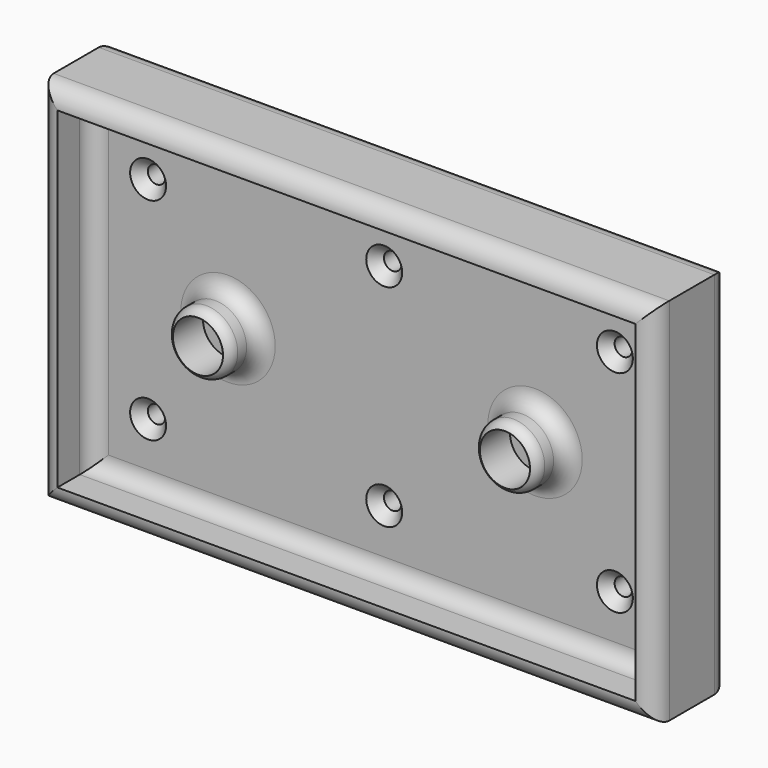
from build123d import *

# Parameters (mm, degrees)
F0_W            = 98.3085063696
F0_H            = 59.0165173113
F0_W_2          = 92.3085063696
F0_H_2          = 53.0165173113
F1_DEPTH        = 8
F2_DEPTH        = 15
F3_R            = 5
F3_R_2          = 4
F4_DEPTH        = 6
F5_R            = 2.54
F6_R            = 3
F7_R            = 2.99999
F10_D           = 2.794
F10_CSINK_D     = 5.7404
F10_CSINK_ANGLE = 82


# Not quite as in the source:
# - a fillet or chamfer that OpenCascade refuses, or shapes differently, is made with other operations: its cross-section is extruded or revolved along the edge and cut away or added
# - a fillet or chamfer is up to 0.001 mm smaller than in the source, because OpenCascade refuses the exact size


with BuildPart() as f1:
    # F0 (on Front) → F1 (new body)
    with BuildSketch(Plane.XZ):
        Rectangle(F0_W, F0_H)
        Rectangle(F0_W_2, F0_H_2, mode=Mode.SUBTRACT)
        Rectangle(F0_W_2, F0_H_2)
    extrude(amount=F1_DEPTH)

    # F0 (on Front) → F2 (join)
    with BuildSketch(Plane.XZ):
        Rectangle(F0_W, F0_H)
        Rectangle(F0_W_2, F0_H_2, mode=Mode.SUBTRACT)
    extrude(amount=F2_DEPTH)

    # F3 (on face) → F4 (join)
    with BuildSketch(Plane.XZ.offset(8)):
        with Locations((-24.5116613805, 0)):
            Circle(F3_R)
        with Locations((-24.5116613805, 0)):
            Circle(F3_R_2, mode=Mode.SUBTRACT)
        with Locations((24.5116613805, 0)):
            Circle(F3_R)
        with Locations((24.5116613805, 0)):
            Circle(F3_R_2, mode=Mode.SUBTRACT)
    extrude(amount=F4_DEPTH)

    # F5
    f5_edges = [f1.edges().sort_by_distance(p)[0] for p in [
        (-29.511661, -8, 0),
        (19.511661, -8, 0),
        (0, -8, -26.508259),
        (46.154253, -8, 0),
        (-46.154253, -8, 0),
        (0, -8, 26.508259),
    ]]
    fillet(f5_edges, radius=F5_R)

    # F6
    f6_edges = [f1.edges().sort_by_distance(p)[0] for p in [
        (0, 0, 29.508259),
        (49.154253, 0, 0),
        (0, 0, -29.508259),
        (-49.154253, 0, 0),
    ]]
    fillet(f6_edges, radius=F6_R)

    # F7 (radius 3 in the source; OpenCascade refuses exactly that, so slightly less here)
    f7_edges = [f1.edges().sort_by_distance(p)[0] for p in [
        (0, -15, -29.508259),
        (49.154253, -15, 0),
        (-49.154253, -15, 0),
        (0, -15, 29.508259),
    ]]
    fillet(f7_edges, radius=F7_R)

    # F8: fillet of radius 2 on 2 edges, made by hand

    # F8_s1 → F8_t2 (revolve, cut)
    with BuildSketch(Plane.XY):
        with BuildLine():
            ThreePointArc((29.5120613805, -12.2673917434), (29.2440686279, -13.2678330874), (28.5118614771, -14.0003463544))
            Line((28.5118614771, -14.0003463544), (28.6119780552, -14.1736418155))
            ThreePointArc((28.6119780552, -14.1736418155), (29.0117614288, -14.2001365685), (29.5116613805, -14.2001365685))
            Line((29.5116613805, -14.2001365685), (29.7117979491, -14))
            ThreePointArc((29.7117979491, -14), (29.7117979491, -13.1336958717), (29.7121979491, -12.2673917434))
            Line((29.7121979491, -12.2673917434), (29.5120613805, -12.2673917434))
        make_face()
    revolve(axis=Axis((24.5116613805, -14, 0), (0, -1, 0)), mode=Mode.SUBTRACT)

    # F8_s3 → F8_t4 (revolve, cut)
    with BuildSketch(Plane.XY):
        with BuildLine():
            ThreePointArc((-19.5112613805, -12.2673917434), (-19.7792541332, -13.2678330874), (-20.511461284, -14.0003463544))
            Line((-20.511461284, -14.0003463544), (-20.4113447058, -14.1736418155))
            ThreePointArc((-20.4113447058, -14.1736418155), (-20.0115613323, -14.2001365685), (-19.5116613805, -14.2001365685))
            Line((-19.5116613805, -14.2001365685), (-19.311524812, -14))
            ThreePointArc((-19.311524812, -14), (-19.311524812, -13.1336958717), (-19.311124812, -12.2673917434))
            Line((-19.311124812, -12.2673917434), (-19.5112613805, -12.2673917434))
        make_face()
    revolve(axis=Axis((-24.5116613805, -14, 0), (0, -1, 0)), mode=Mode.SUBTRACT)

    # F10 (through all)
    with Locations(Plane.XZ.offset(8)):
        with Locations((37.2699052095, 16.8491732329), (37.2699052095, -16.8491732329), (0.4332323442, -16.7640619911), (0.4332323442, 16.9342844747), (-37.2699052095, 16.8491732329), (-37.2699052095, -16.8491732329)):
            CounterSinkHole(F10_D / 2, F10_CSINK_D / 2, counter_sink_angle=F10_CSINK_ANGLE)


solid = f1.part
